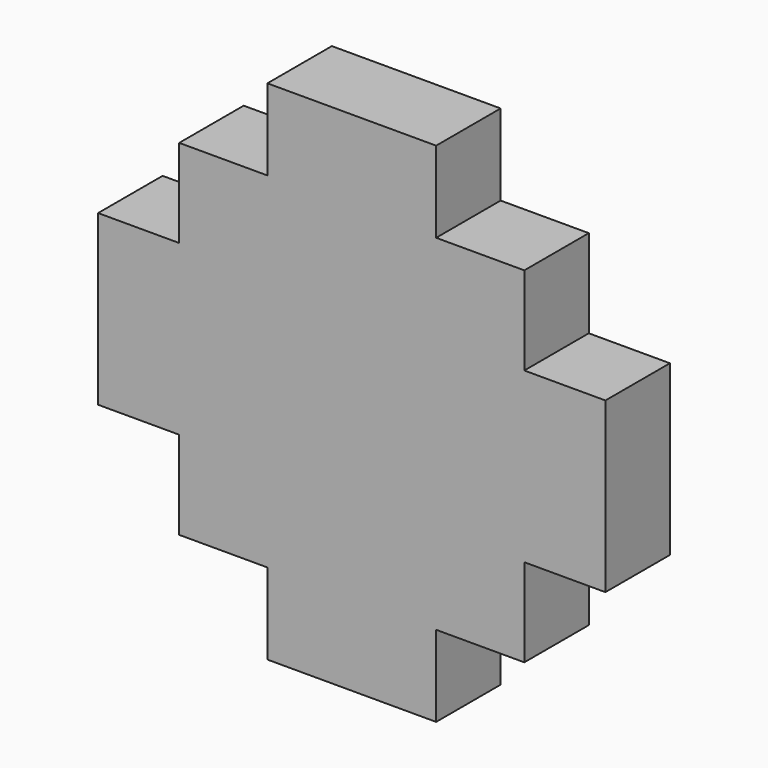
from build123d import *

# Parameters (mm, degrees)
F1_DEPTH     = 2.032
F2_TEXT_SIZE = 9.4030674849
F3_DEPTH     = 0.508


# Not quite as in the source:
# - Text() gives the source's letters only with a copy of the font that has no kerning and outlines rounded to 1/6400 em; it was checked with that copy


with BuildPart() as f1:
    # F0 (on Front) → F1 (new body)
    with BuildSketch(Plane.XZ):
        Polygon((-15.2212520439, 36.2265945869), (-17.3485020439, 36.2265945869), (-19.4757520439, 36.2265945869), (-19.4757520439, 34.1818945869), (-21.6982520439, 34.1818945869), (-21.6982520439, 31.9593945869), (-23.7429520439, 31.9593945869), (-23.7429520439, 29.8321445869), (-23.7429520439, 27.7048945869), (-21.6982520439, 27.7048945869), (-21.6982520439, 25.4823945869), (-19.4757520439, 25.4823945869), (-19.4757520439, 23.4376945869), (-17.3485020439, 23.4376945869), (-15.2212520439, 23.4376945869), (-15.2212520439, 25.4823945869), (-12.9987520439, 25.4823945869), (-12.9987520439, 27.7048945869), (-10.9540520439, 27.7048945869), (-10.9540520439, 29.8321445869), (-10.9540520439, 31.9593945869), (-12.9987520439, 31.9593945869), (-12.9987520439, 34.1818945869), (-15.2212520439, 34.1818945869), align=None)
    extrude(amount=F1_DEPTH)

    # F2 (on Front) → F3 (cut)
    with BuildSketch(Plane.XZ):
        with Locations((-20.6340369446, 26.2480336348)):
            Text('A', F2_TEXT_SIZE, font='Open Sans', text_align=(TextAlign.LEFT, TextAlign.BOTTOM))
    extrude(amount=F3_DEPTH, mode=Mode.SUBTRACT)


solid = f1.part
